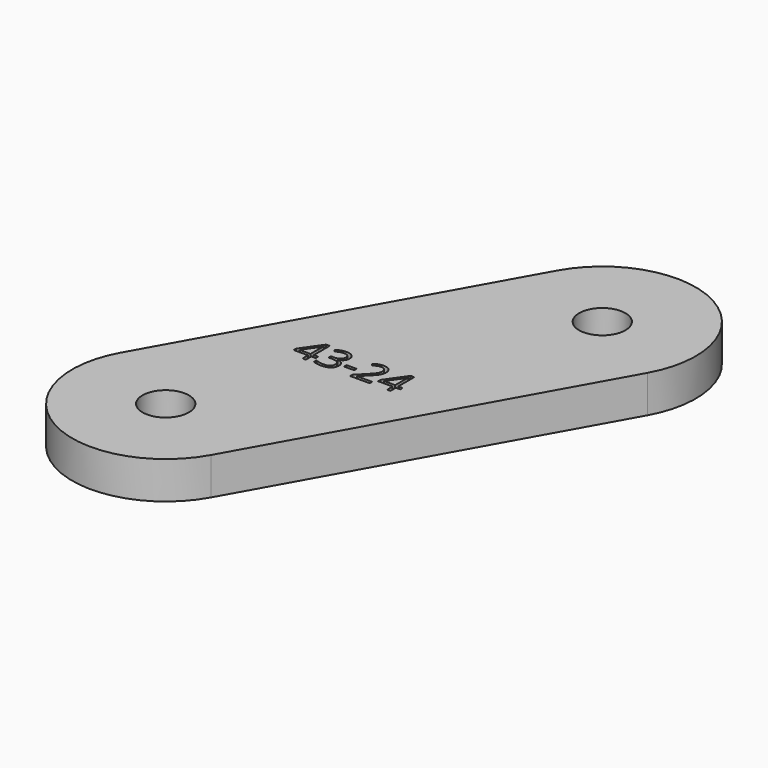
from build123d import *

# Parameters (mm, degrees)
F1_R         = 3.1
F2_DEPTH     = 5
F3_TEXT_SIZE = 5.5555555556
F4_DEPTH     = 2


# Not quite as in the source:
# - Text() gives the source's letters only with a copy of the font that has no kerning and outlines rounded to 1/6400 em; it was checked with that copy


with BuildPart() as f2:
    # F1 (on Top) → F2 (new body)
    with BuildSketch(Plane.XY):
        with BuildLine():
            Line((13.0850287248, 49.0920769908), (-10.9149712752, 6.0920769908))
            ThreePointArc((-10.9149712752, 6.0920769908), (-6.0920769908, -10.9149712752), (10.9149712752, -6.0920769908))
            Line((10.9149712752, -6.0920769908), (34.9149712752, 36.9079230092))
            ThreePointArc((34.9149712752, 36.9079230092), (30.0920769908, 53.9149712752), (13.0850287248, 49.0920769908))
        make_face()
        Circle(F1_R, mode=Mode.SUBTRACT)
        with Locations((24, 43)):
            Circle(F1_R, mode=Mode.SUBTRACT)
    extrude(amount=F2_DEPTH)

    # F3 (on face) → F4 (cut)
    with BuildSketch(Plane.XY.offset(5)):
        with Locations((2.707536411, 16.9472606985)):
            Text('43-24', F3_TEXT_SIZE, font='Open Sans', text_align=(TextAlign.LEFT, TextAlign.BOTTOM))
    extrude(amount=-F4_DEPTH, mode=Mode.SUBTRACT)


solid = f2.part
